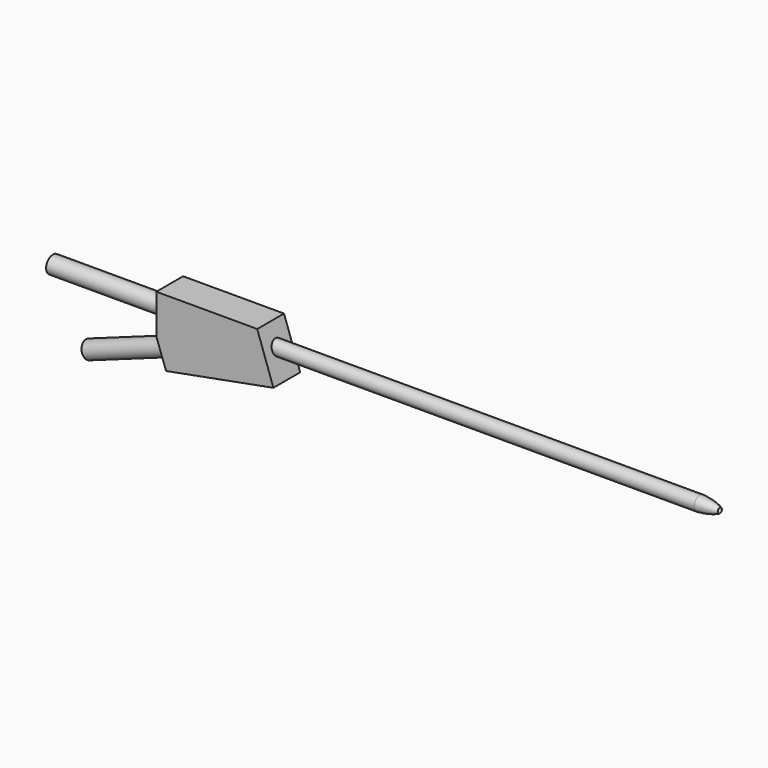
from build123d import *

# Parameters (mm, degrees)
F3_DEPTH       = 2.4765
F4_R           = 1.27
F5_DEPTH       = 17.272
F6_R           = 1.27
F7_DEPTH       = 13.462
F8_R           = 1.0434793425
F9_DEPTH       = 95.7072
F9_DEPTH_BACK  = 132
F10_R          = 0.3833262894
F11_DEPTH      = 32.2036075046
F11_DEPTH_BACK = 66.8030001


# Not quite as in the source:
# - an extrude ends at something that could not be found from the text; its depth is read off the source's solid


with BuildPart() as f1:
    # F0 (on Front) → F1 (revolve)
    with BuildSketch(Plane.XZ):
        with BuildLine():
            Line((63.5, 1.0541), (0, 1.0541))
            Line((0, 1.0541), (0, 0))
            Line((0, 0), (66.802, 0))
            add(Edge.make_bspline(
                [(63.5, 1.0541), (64.35611099, 1.0419137543), (66.7864059348, 0.5992812803), (66.802, 0)],
                knots=[0, 0, 0, 0, 3.4661694722, 3.4661694722, 3.4661694722, 3.4661694722], degree=3))
        make_face()
    revolve(axis=Axis((33.401, 0, 0), (1, 0, 0)))

    # F2 (on Front) → F3 (join, symmetric)
    with BuildSketch(Plane.XZ):
        Polygon((0.0045924954, 3.0420540417), (-14.9306075046, 3.0420540417), (-14.9306075046, -2.7999459583), (-13.4860288486, -6.8151904523), (2.3921924954, -3.8408457662), align=None)
    extrude(amount=F3_DEPTH, both=True)

    # F4 (on face) → F5 (join)
    with BuildSketch(Plane(origin=(-14.9306075046, 0, 0), x_dir=(0, -1, 0), z_dir=(-1, 0, 0))):
        Circle(F4_R)
    extrude(amount=F5_DEPTH)

    # F6 (on face) → F7 (join)
    with BuildSketch(Plane(origin=(-14.1114148908, 0, -5.0769134453), x_dir=(0, -1, 0), z_dir=(-0.9409553089, 0, -0.3385308062))):
        with Locations((0, 0.2862465809)):
            Circle(F6_R)
    extrude(amount=F7_DEPTH)

    # F8 (on face) → F9 (cut, two sides)
    with BuildSketch(Plane(origin=(-32.2026075046, 0, 0), x_dir=(0, -1, 0), z_dir=(-1, 0, 0))) as f9_sk:
        Circle(F8_R)
    extrude(amount=-F9_DEPTH, mode=Mode.SUBTRACT)
    extrude(f9_sk.sketch, amount=F9_DEPTH_BACK, mode=Mode.SUBTRACT)

    # F10 (on Right) → F11 (cut, two sides)
    with BuildSketch(Plane.YZ) as f11_sk:
        Circle(F10_R)
    extrude(amount=-F11_DEPTH, mode=Mode.SUBTRACT)
    extrude(f11_sk.sketch, amount=F11_DEPTH_BACK, mode=Mode.SUBTRACT)


solid = f1.part
